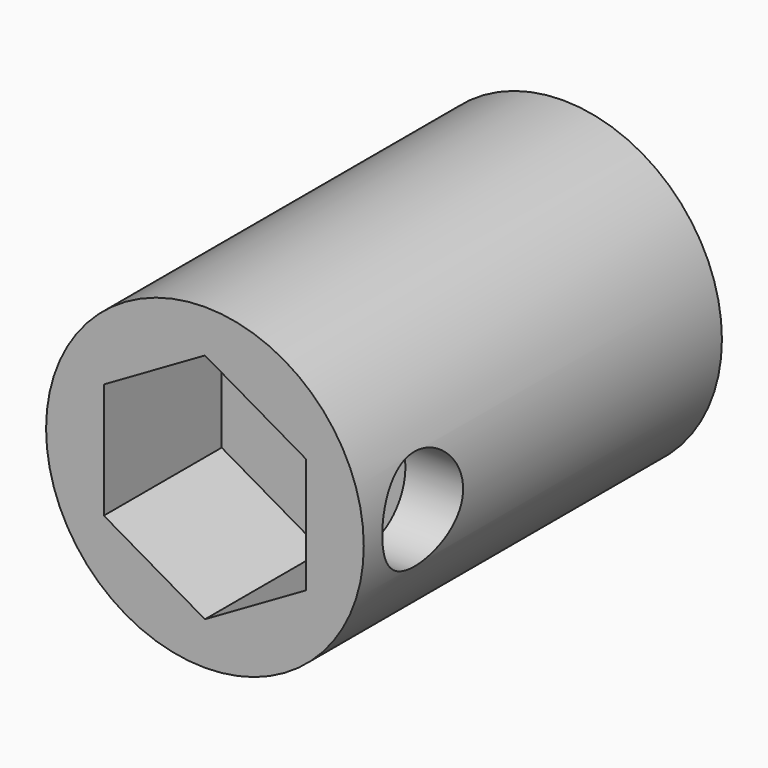
from build123d import *

# Parameters (mm, degrees)
F0_R      = 5.5
F1_DEPTH  = 15.5
F2_R      = 1.5
F3_DEPTH  = 9
F5_R      = 1.25
F6_DEPTH  = 6
F4_R      = 1.5
F7_DEPTH  = 5.1
F9_DEPTH  = 25.4
F11_ANGLE = 180
F13_ANGLE = -90
F15_ANGLE = 90


# Not quite as in the source:
# - a feature names something its author has since deleted; it is built from what else it names


with BuildPart() as f1:
    # F0 (on Top) → F1 (new body)
    with BuildSketch(Plane.XY):
        Circle(F0_R)
    extrude(amount=F1_DEPTH)

    # F2 (on face) → F3 (cut)
    with BuildSketch(Plane(origin=(0, 0, 0), x_dir=(1, 0, 0), z_dir=(0, 0, -1))):
        Circle(F2_R)
    extrude(amount=-F3_DEPTH, mode=Mode.SUBTRACT)

    # F5 (on face) → F6 (cut)
    with BuildSketch(Plane.XY.offset(15.5)):
        Circle(F5_R)
    extrude(amount=-F6_DEPTH, mode=Mode.SUBTRACT)

    # F4 (on face) → F7 (cut)
    with BuildSketch(Plane(origin=(0, 0, 0), x_dir=(1, 0, 0), z_dir=(0, 0, -1))):
        Polygon((2, 3.5), (-2, 3.5), (-4.0207259422, 0), (-2, -3.5), (2, -3.5), (4.0207259422, 0), align=None)
        Circle(F4_R, mode=Mode.SUBTRACT)
    extrude(amount=-F7_DEPTH, mode=Mode.SUBTRACT)

    # F8 (on face) → F9 (cut)
    with BuildSketch(Plane.XZ.offset(-3.5)):
        with BuildLine():
            ThreePointArc((1.75, 2.55), (-1.2374368671, 3.7874368671), (0, 0.8))
            ThreePointArc((0, 0.8), (1.2374368671, 1.3125631329), (1.75, 2.55))
        make_face()
    extrude(amount=-F9_DEPTH, mode=Mode.SUBTRACT)


with BuildPart() as f1_1:
    # F11: moved
    add(f1.part.rotate(Axis((9.4123384915, 0, 0), (1, 0, 0)), F11_ANGLE))


with BuildPart() as f1_2:
    # F13: moved
    add(f1_1.part.rotate(Axis((-2.3788576946, 0, 0), (-1, 0, 0)), F13_ANGLE))


with BuildPart() as f1_3:
    # F15: moved
    add(f1_2.part.rotate(Axis((0, 5.9970328584, 0), (0, -1, 0)), F15_ANGLE))


solid = f1_3.part
